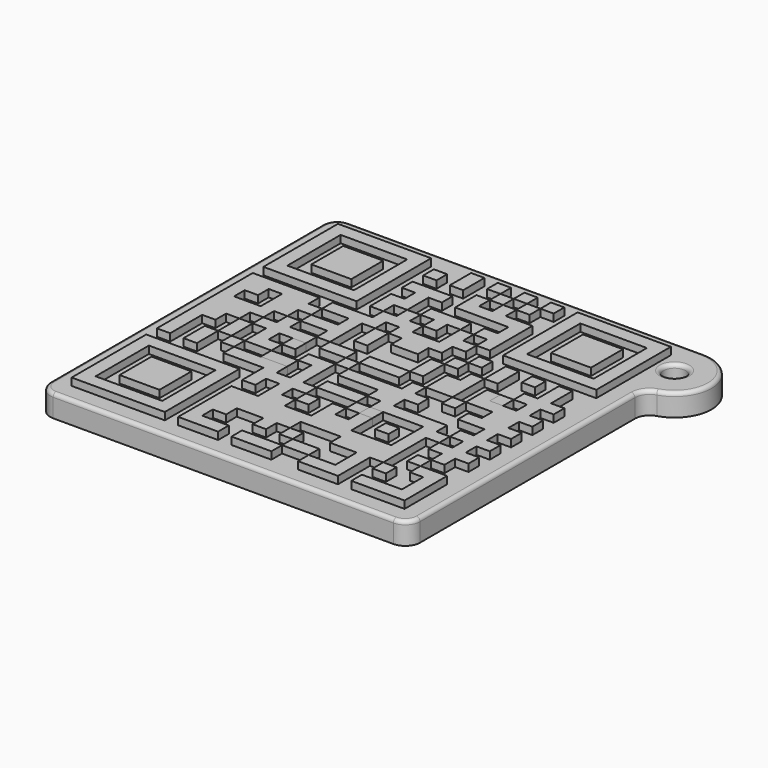
from build123d import *

# Parameters (mm, degrees)
F0_R     = 1.5
F1_DEPTH = 3
F2_R     = 2
F3_W     = 1.8
F3_H     = 1.8
F4_DEPTH = 1
F5_W     = 1.8
F5_H     = 1.8
F6_DEPTH = 1
F5_W_2   = 3.6
F7_R     = 0.5


with BuildPart() as f1:
    # F0 (on Top) → F1 (new body)
    with BuildSketch(Plane.XY):
        with BuildLine():
            Line((25, 25), (-25, 25))
            Line((-25, 25), (-25, -25))
            Line((-25, -25), (25, -25))
            Line((25, -25), (25, 15))
            ThreePointArc((25, 15), (30, 20), (25, 25))
        make_face()
        with Locations((25, 20)):
            Circle(F0_R, mode=Mode.SUBTRACT)
    extrude(amount=-F1_DEPTH)

    # F2
    f2_edges = [f1.edges().sort_by_distance(p)[0] for p in [
        (-25, -25, -1.5),
        (25, -25, -1.5),
        (25, 15, -1.5),
        (-25, 25, -1.5),
    ]]
    fillet(f2_edges, radius=F2_R)

    # F7
    f7_edges = [f1.edges().sort_by_distance(p)[0] for p in [
        (23.5, 20, 0),
        (23.5, 20, -3),
        (1, 25, 0),
    ]]
    fillet(f7_edges, radius=F7_R)


with BuildPart() as f4:
    # F3 (on Top) → F4 (new body)
    with BuildSketch(Plane.XY):
        with Locations((21.5957503378, 21.6023441762)):
            Rectangle(F3_W, F3_H)
        with Locations((21.5957503378, 19.8023441762)):
            Rectangle(F3_W, F3_H)
        with Locations((21.5957503378, 18.0023441762)):
            Rectangle(F3_W, F3_H)
        with Locations((21.5957503378, 16.2023441762)):
            Rectangle(F3_W, F3_H)
        with Locations((21.5957503378, 14.4023441762)):
            Rectangle(F3_W, F3_H)
        with Locations((21.5957503378, 12.6023441762)):
            Rectangle(F3_W, F3_H)
        with Locations((21.5957503378, 10.8023441762)):
            Rectangle(F3_W, F3_H)
        with Locations((19.7957503378, 21.6023441762)):
            Rectangle(F3_W, F3_H)
        with Locations((17.9957503378, 21.6023441762)):
            Rectangle(F3_W, F3_H)
        with Locations((16.1957503378, 21.6023441762)):
            Rectangle(F3_W, F3_H)
        with Locations((14.3957503378, 21.6023441762)):
            Rectangle(F3_W, F3_H)
        with Locations((12.5957503378, 21.6023441762)):
            Rectangle(F3_W, F3_H)
        with Locations((10.7957503378, 21.6023441762)):
            Rectangle(F3_W, F3_H)
        with Locations((10.7957503378, 19.8023441762)):
            Rectangle(F3_W, F3_H)
        with Locations((10.7957503378, 18.0023441762)):
            Rectangle(F3_W, F3_H)
        with Locations((10.7957503378, 16.2023441762)):
            Rectangle(F3_W, F3_H)
        with Locations((10.7957503378, 14.4023441762)):
            Rectangle(F3_W, F3_H)
        with Locations((10.7957503378, 12.6023441762)):
            Rectangle(F3_W, F3_H)
        with Locations((10.7957503378, 10.8023441762)):
            Rectangle(F3_W, F3_H)
        with Locations((12.5957503378, 10.8023441762)):
            Rectangle(F3_W, F3_H)
        with Locations((14.3957503378, 10.8023441762)):
            Rectangle(F3_W, F3_H)
        with Locations((16.1957503378, 10.8023441762)):
            Rectangle(F3_W, F3_H)
        with Locations((17.9957503378, 10.8023441762)):
            Rectangle(F3_W, F3_H)
        with Locations((19.7957503378, 10.8023441762)):
            Rectangle(F3_W, F3_H)
    extrude(amount=F4_DEPTH)


with BuildPart() as f4b:
    # F3 (on Top) → F4, piece 2 (new body)
    with BuildSketch(Plane.XY):
        with Locations((21.5957503378, -21.5976558238)):
            Rectangle(F3_W, F3_H)
        with Locations((21.5957503378, -16.1976558238)):
            Rectangle(F3_W, F3_H)
        with Locations((21.5957503378, -17.9976558238)):
            Rectangle(F3_W, F3_H)
        with Locations((21.5957503378, -19.7976558238)):
            Rectangle(F3_W, F3_H)
        with Locations((19.7957503378, -21.5976558238)):
            Rectangle(F3_W, F3_H)
        with Locations((17.9957503378, -21.5976558238)):
            Rectangle(F3_W, F3_H)
        with Locations((16.1957503378, -21.5976558238)):
            Rectangle(F3_W, F3_H)
        with Locations((19.7957503378, -16.1976558238)):
            Rectangle(F3_W, F3_H)
    extrude(amount=F4_DEPTH)


with BuildPart() as f4c:
    # F3 (on Top) → F4, piece 3 (new body)
    with BuildSketch(Plane.XY):
        with Locations((-21.6042496622, 21.6023441762)):
            Rectangle(F3_W, F3_H)
        with Locations((-10.8042496622, 21.6023441762)):
            Rectangle(F3_W, F3_H)
        with Locations((-12.6042496622, 21.6023441762)):
            Rectangle(F3_W, F3_H)
        with Locations((-14.4042496622, 21.6023441762)):
            Rectangle(F3_W, F3_H)
        with Locations((-16.2042496622, 21.6023441762)):
            Rectangle(F3_W, F3_H)
        with Locations((-18.0042496622, 21.6023441762)):
            Rectangle(F3_W, F3_H)
        with Locations((-19.8042496622, 21.6023441762)):
            Rectangle(F3_W, F3_H)
        with Locations((-21.6042496622, 19.8023441762)):
            Rectangle(F3_W, F3_H)
        with Locations((-21.6042496622, 18.0023441762)):
            Rectangle(F3_W, F3_H)
        with Locations((-21.6042496622, 16.2023441762)):
            Rectangle(F3_W, F3_H)
        with Locations((-21.6042496622, 14.4023441762)):
            Rectangle(F3_W, F3_H)
        with Locations((-21.6042496622, 12.6023441762)):
            Rectangle(F3_W, F3_H)
        with Locations((-21.6042496622, 10.8023441762)):
            Rectangle(F3_W, F3_H)
        with Locations((-19.8042496622, 10.8023441762)):
            Rectangle(F3_W, F3_H)
        with Locations((-18.0042496622, 10.8023441762)):
            Rectangle(F3_W, F3_H)
        with Locations((-16.2042496622, 10.8023441762)):
            Rectangle(F3_W, F3_H)
        with Locations((-14.4042496622, 10.8023441762)):
            Rectangle(F3_W, F3_H)
        with Locations((-12.6042496622, 10.8023441762)):
            Rectangle(F3_W, F3_H)
        with Locations((-10.8042496622, 10.8023441762)):
            Rectangle(F3_W, F3_H)
        with Locations((-10.8042496622, 12.6023441762)):
            Rectangle(F3_W, F3_H)
        with Locations((-10.8042496622, 14.4023441762)):
            Rectangle(F3_W, F3_H)
        with Locations((-10.8042496622, 16.2023441762)):
            Rectangle(F3_W, F3_H)
        with Locations((-10.8042496622, 18.0023441762)):
            Rectangle(F3_W, F3_H)
        with Locations((-10.8042496622, 19.8023441762)):
            Rectangle(F3_W, F3_H)
    extrude(amount=F4_DEPTH)


with BuildPart() as f4d:
    # F3 (on Top) → F4, piece 4 (new body)
    with BuildSketch(Plane.XY):
        with Locations((-21.6042496622, -21.5976558238)):
            Rectangle(F3_W, F3_H)
        with Locations((-10.8042496622, -21.5976558238)):
            Rectangle(F3_W, F3_H)
        with Locations((-12.6042496622, -21.5976558238)):
            Rectangle(F3_W, F3_H)
        with Locations((-14.4042496622, -21.5976558238)):
            Rectangle(F3_W, F3_H)
        with Locations((-16.2042496622, -21.5976558238)):
            Rectangle(F3_W, F3_H)
        with Locations((-18.0042496622, -21.5976558238)):
            Rectangle(F3_W, F3_H)
        with Locations((-19.8042496622, -21.5976558238)):
            Rectangle(F3_W, F3_H)
        with Locations((-21.6042496622, -10.7976558238)):
            Rectangle(F3_W, F3_H)
        with Locations((-21.6042496622, -12.5976558238)):
            Rectangle(F3_W, F3_H)
        with Locations((-21.6042496622, -14.3976558238)):
            Rectangle(F3_W, F3_H)
        with Locations((-21.6042496622, -16.1976558238)):
            Rectangle(F3_W, F3_H)
        with Locations((-21.6042496622, -17.9976558238)):
            Rectangle(F3_W, F3_H)
        with Locations((-21.6042496622, -19.7976558238)):
            Rectangle(F3_W, F3_H)
        with Locations((-19.8042496622, -10.7976558238)):
            Rectangle(F3_W, F3_H)
        with Locations((-18.0042496622, -10.7976558238)):
            Rectangle(F3_W, F3_H)
        with Locations((-16.2042496622, -10.7976558238)):
            Rectangle(F3_W, F3_H)
        with Locations((-14.4042496622, -10.7976558238)):
            Rectangle(F3_W, F3_H)
        with Locations((-12.6042496622, -10.7976558238)):
            Rectangle(F3_W, F3_H)
        with Locations((-10.8042496622, -10.7976558238)):
            Rectangle(F3_W, F3_H)
        with Locations((-10.8042496622, -12.5976558238)):
            Rectangle(F3_W, F3_H)
        with Locations((-10.8042496622, -14.3976558238)):
            Rectangle(F3_W, F3_H)
        with Locations((-10.8042496622, -16.1976558238)):
            Rectangle(F3_W, F3_H)
        with Locations((-10.8042496622, -17.9976558238)):
            Rectangle(F3_W, F3_H)
        with Locations((-10.8042496622, -19.7976558238)):
            Rectangle(F3_W, F3_H)
    extrude(amount=F4_DEPTH)


with BuildPart() as f4e:
    # F3 (on Top) → F4, piece 5 (new body)
    with BuildSketch(Plane.XY):
        with Locations((21.5957503378, 3.6023441762)):
            Rectangle(F3_W, F3_H)
        with Locations((21.5957503378, 0.0023441762)):
            Rectangle(F3_W, F3_H)
        with Locations((21.5957503378, -3.5976558238)):
            Rectangle(F3_W, F3_H)
        with Locations((21.5957503378, -7.1976558238)):
            Rectangle(F3_W, F3_H)
        with Locations((21.5957503378, -10.7976558238)):
            Rectangle(F3_W, F3_H)
        with Locations((19.7957503378, -12.5976558238)):
            Rectangle(F3_W, F3_H)
        with Locations((19.7957503378, -10.7976558238)):
            Rectangle(F3_W, F3_H)
        with Locations((19.7957503378, -8.9976558238)):
            Rectangle(F3_W, F3_H)
        with Locations((19.7957503378, -7.1976558238)):
            Rectangle(F3_W, F3_H)
        with Locations((19.7957503378, -5.3976558238)):
            Rectangle(F3_W, F3_H)
        with Locations((19.7957503378, -3.5976558238)):
            Rectangle(F3_W, F3_H)
        with Locations((17.9957503378, -10.7976558238)):
            Rectangle(F3_W, F3_H)
        with Locations((17.9957503378, -7.1976558238)):
            Rectangle(F3_W, F3_H)
        with Locations((16.1957503378, -3.5976558238)):
            Rectangle(F3_W, F3_H)
        with Locations((17.9957503378, -3.5976558238)):
            Rectangle(F3_W, F3_H)
        with Locations((17.9957503378, -1.7976558238)):
            Rectangle(F3_W, F3_H)
        with Locations((19.7957503378, -1.7976558238)):
            Rectangle(F3_W, F3_H)
        with Locations((19.7957503378, 7.2023441762)):
            Rectangle(F3_W, F3_H)
        with Locations((19.7957503378, 5.4023441762)):
            Rectangle(F3_W, F3_H)
        with Locations((19.7957503378, 3.6023441762)):
            Rectangle(F3_W, F3_H)
        with Locations((17.9957503378, 3.6023441762)):
            Rectangle(F3_W, F3_H)
        with Locations((19.7957503378, 1.8023441762)):
            Rectangle(F3_W, F3_H)
        with Locations((19.7957503378, 0.0023441762)):
            Rectangle(F3_W, F3_H)
        with Locations((17.9957503378, 0.0023441762)):
            Rectangle(F3_W, F3_H)
        with Locations((14.3957503378, 0.0023441762)):
            Rectangle(F3_W, F3_H)
        with Locations((16.1957503378, 0.0023441762)):
            Rectangle(F3_W, F3_H)
        with Locations((14.3957503378, 1.8023441762)):
            Rectangle(F3_W, F3_H)
    extrude(amount=F4_DEPTH)


with BuildPart() as f4f:
    # F3 (on Top) → F4, piece 6 (new body)
    with BuildSketch(Plane.XY):
        with Locations((12.5957503378, -21.5976558238)):
            Rectangle(F3_W, F3_H)
        with Locations((10.7957503378, -21.5976558238)):
            Rectangle(F3_W, F3_H)
        with Locations((8.9957503378, -21.5976558238)):
            Rectangle(F3_W, F3_H)
        with Locations((-3.6042496622, -21.5976558238)):
            Rectangle(F3_W, F3_H)
        with Locations((-5.4042496622, -21.5976558238)):
            Rectangle(F3_W, F3_H)
        with Locations((-7.2042496622, -21.5976558238)):
            Rectangle(F3_W, F3_H)
        with Locations((-12.6042496622, -7.1976558238)):
            Rectangle(F3_W, F3_H)
        with Locations((-10.8042496622, -7.1976558238)):
            Rectangle(F3_W, F3_H)
        with Locations((12.5957503378, -19.7976558238)):
            Rectangle(F3_W, F3_H)
        with Locations((12.5957503378, -17.9976558238)):
            Rectangle(F3_W, F3_H)
        with Locations((-7.2042496622, -19.7976558238)):
            Rectangle(F3_W, F3_H)
        with Locations((-7.2042496622, -17.9976558238)):
            Rectangle(F3_W, F3_H)
        with Locations((-5.4042496622, -17.9976558238)):
            Rectangle(F3_W, F3_H)
        with Locations((-0.0042496622, -17.9976558238)):
            Rectangle(F3_W, F3_H)
        with Locations((-7.2042496622, -16.1976558238)):
            Rectangle(F3_W, F3_H)
        with Locations((-5.4042496622, -16.1976558238)):
            Rectangle(F3_W, F3_H)
        with Locations((-3.6042496622, -16.1976558238)):
            Rectangle(F3_W, F3_H)
        with Locations((-1.8042496622, -16.1976558238)):
            Rectangle(F3_W, F3_H)
        with Locations((-0.0042496622, -16.1976558238)):
            Rectangle(F3_W, F3_H)
        with Locations((1.7957503378, -16.1976558238)):
            Rectangle(F3_W, F3_H)
        with Locations((8.9957503378, -16.1976558238)):
            Rectangle(F3_W, F3_H)
        with Locations((10.7957503378, -16.1976558238)):
            Rectangle(F3_W, F3_H)
        with Locations((12.5957503378, -16.1976558238)):
            Rectangle(F3_W, F3_H)
        with Locations((14.3957503378, -16.1976558238)):
            Rectangle(F3_W, F3_H)
        with Locations((14.3957503378, -7.1976558238)):
            Rectangle(F3_W, F3_H)
        with Locations((14.3957503378, -8.9976558238)):
            Rectangle(F3_W, F3_H)
        with Locations((16.1957503378, -8.9976558238)):
            Rectangle(F3_W, F3_H)
        with Locations((14.3957503378, -10.7976558238)):
            Rectangle(F3_W, F3_H)
        with Locations((14.3957503378, -12.5976558238)):
            Rectangle(F3_W, F3_H)
        with Locations((14.3957503378, -14.3976558238)):
            Rectangle(F3_W, F3_H)
        with Locations((12.5957503378, -14.3976558238)):
            Rectangle(F3_W, F3_H)
        with Locations((10.7957503378, -14.3976558238)):
            Rectangle(F3_W, F3_H)
        with Locations((8.9957503378, -14.3976558238)):
            Rectangle(F3_W, F3_H)
        with Locations((-7.2042496622, -14.3976558238)):
            Rectangle(F3_W, F3_H)
        with Locations((-5.4042496622, -14.3976558238)):
            Rectangle(F3_W, F3_H)
        with Locations((-3.6042496622, -14.3976558238)):
            Rectangle(F3_W, F3_H)
        with Locations((-1.8042496622, -14.3976558238)):
            Rectangle(F3_W, F3_H)
        with Locations((-0.0042496622, -14.3976558238)):
            Rectangle(F3_W, F3_H)
        with Locations((1.7957503378, -14.3976558238)):
            Rectangle(F3_W, F3_H)
        with Locations((3.5957503378, -14.3976558238)):
            Rectangle(F3_W, F3_H)
        with Locations((5.3957503378, -14.3976558238)):
            Rectangle(F3_W, F3_H)
        with Locations((7.1957503378, -14.3976558238)):
            Rectangle(F3_W, F3_H)
        with Locations((7.1957503378, -12.5976558238)):
            Rectangle(F3_W, F3_H)
        with Locations((5.3957503378, -12.5976558238)):
            Rectangle(F3_W, F3_H)
        with Locations((3.5957503378, -12.5976558238)):
            Rectangle(F3_W, F3_H)
        with Locations((-1.8042496622, -12.5976558238)):
            Rectangle(F3_W, F3_H)
        with Locations((-3.6042496622, -12.5976558238)):
            Rectangle(F3_W, F3_H)
        with Locations((-7.2042496622, -10.7976558238)):
            Rectangle(F3_W, F3_H)
        with Locations((-3.6042496622, -10.7976558238)):
            Rectangle(F3_W, F3_H)
        with Locations((3.5957503378, -10.7976558238)):
            Rectangle(F3_W, F3_H)
        with Locations((7.1957503378, -10.7976558238)):
            Rectangle(F3_W, F3_H)
        with Locations((-7.2042496622, -8.9976558238)):
            Rectangle(F3_W, F3_H)
        with Locations((-5.4042496622, -8.9976558238)):
            Rectangle(F3_W, F3_H)
        with Locations((-3.6042496622, -8.9976558238)):
            Rectangle(F3_W, F3_H)
        with Locations((-1.8042496622, -8.9976558238)):
            Rectangle(F3_W, F3_H)
        with Locations((-5.4042496622, -3.5976558238)):
            Rectangle(F3_W, F3_H)
        with Locations((-3.6042496622, -3.5976558238)):
            Rectangle(F3_W, F3_H)
        with Locations((-3.6042496622, -5.3976558238)):
            Rectangle(F3_W, F3_H)
        with Locations((-3.6042496622, -7.1976558238)):
            Rectangle(F3_W, F3_H)
        with Locations((-0.0042496622, -3.5976558238)):
            Rectangle(F3_W, F3_H)
        with Locations((1.7957503378, -3.5976558238)):
            Rectangle(F3_W, F3_H)
        with Locations((3.5957503378, -3.5976558238)):
            Rectangle(F3_W, F3_H)
        with Locations((5.3957503378, -3.5976558238)):
            Rectangle(F3_W, F3_H)
        with Locations((8.9957503378, -3.5976558238)):
            Rectangle(F3_W, F3_H)
        with Locations((5.3957503378, -5.3976558238)):
            Rectangle(F3_W, F3_H)
        with Locations((7.1957503378, -5.3976558238)):
            Rectangle(F3_W, F3_H)
        with Locations((7.1957503378, -3.5976558238)):
            Rectangle(F3_W, F3_H)
        with Locations((7.1957503378, -1.7976558238)):
            Rectangle(F3_W, F3_H)
        with Locations((7.1957503378, -7.1976558238)):
            Rectangle(F3_W, F3_H)
        with Locations((8.9957503378, -7.1976558238)):
            Rectangle(F3_W, F3_H)
        with Locations((10.7957503378, -7.1976558238)):
            Rectangle(F3_W, F3_H)
        with Locations((12.5957503378, -7.1976558238)):
            Rectangle(F3_W, F3_H)
        with Locations((-7.2042496622, -7.1976558238)):
            Rectangle(F3_W, F3_H)
        with Locations((-9.0042496622, -7.1976558238)):
            Rectangle(F3_W, F3_H)
    extrude(amount=F4_DEPTH)


with BuildPart() as f4g:
    # F3 (on Top) → F4, piece 7 (new body)
    with BuildSketch(Plane.XY):
        with Locations((3.5957503378, -21.5976558238)):
            Rectangle(F3_W, F3_H)
        with Locations((1.7957503378, -21.5976558238)):
            Rectangle(F3_W, F3_H)
        with Locations((-0.0042496622, -21.5976558238)):
            Rectangle(F3_W, F3_H)
    extrude(amount=F4_DEPTH)


with BuildPart() as f4h:
    # F3 (on Top) → F4, piece 8 (new body)
    with BuildSketch(Plane.XY):
        with Locations((-3.6042496622, 21.6023441762)):
            Rectangle(F3_W, F3_H)
        with Locations((-3.6042496622, 19.8023441762)):
            Rectangle(F3_W, F3_H)
    extrude(amount=F4_DEPTH)


with BuildPart() as f4i:
    # F3 (on Top) → F4, piece 9 (new body)
    with BuildSketch(Plane.XY):
        with Locations((-21.6042496622, 7.2023441762)):
            Rectangle(F3_W, F3_H)
        with Locations((-21.6042496622, 5.4023441762)):
            Rectangle(F3_W, F3_H)
        with Locations((-21.6042496622, 3.6023441762)):
            Rectangle(F3_W, F3_H)
        with Locations((-21.6042496622, 1.8023441762)):
            Rectangle(F3_W, F3_H)
        with Locations((-21.6042496622, 0.0023441762)):
            Rectangle(F3_W, F3_H)
        with Locations((-21.6042496622, -1.7976558238)):
            Rectangle(F3_W, F3_H)
        with Locations((-21.6042496622, -3.5976558238)):
            Rectangle(F3_W, F3_H)
        with Locations((-21.6042496622, -5.3976558238)):
            Rectangle(F3_W, F3_H)
        with Locations((-21.6042496622, -7.1976558238)):
            Rectangle(F3_W, F3_H)
        with Locations((-19.8042496622, -1.7976558238)):
            Rectangle(F3_W, F3_H)
        with Locations((-19.8042496622, 0.0023441762)):
            Rectangle(F3_W, F3_H)
        with Locations((-19.8042496622, 1.8023441762)):
            Rectangle(F3_W, F3_H)
        with Locations((-18.0042496622, 0.0023441762)):
            Rectangle(F3_W, F3_H)
        with Locations((-18.0042496622, 1.8023441762)):
            Rectangle(F3_W, F3_H)
        with Locations((-16.2042496622, 1.8023441762)):
            Rectangle(F3_W, F3_H)
        with Locations((-12.6042496622, 5.4023441762)):
            Rectangle(F3_W, F3_H)
        with Locations((-14.4042496622, 5.4023441762)):
            Rectangle(F3_W, F3_H)
        with Locations((-16.2042496622, 5.4023441762)):
            Rectangle(F3_W, F3_H)
        with Locations((-14.4042496622, 7.2023441762)):
            Rectangle(F3_W, F3_H)
        with Locations((-19.8042496622, 5.4023441762)):
            Rectangle(F3_W, F3_H)
        with Locations((-19.8042496622, 7.2023441762)):
            Rectangle(F3_W, F3_H)
        with Locations((-18.0042496622, 7.2023441762)):
            Rectangle(F3_W, F3_H)
        with Locations((-16.2042496622, 7.2023441762)):
            Rectangle(F3_W, F3_H)
        with Locations((-16.2042496622, 3.6023441762)):
            Rectangle(F3_W, F3_H)
        with Locations((-14.4042496622, 3.6023441762)):
            Rectangle(F3_W, F3_H)
    extrude(amount=F4_DEPTH)


with BuildPart() as f4j:
    # F3 (on Top) → F4, piece 10 (new body)
    with BuildSketch(Plane.XY):
        with Locations((-18.0042496622, 18.0023441762)):
            Rectangle(F3_W, F3_H)
        with Locations((-16.2042496622, 18.0023441762)):
            Rectangle(F3_W, F3_H)
        with Locations((-14.4042496622, 18.0023441762)):
            Rectangle(F3_W, F3_H)
        with Locations((-14.4042496622, 16.2023441762)):
            Rectangle(F3_W, F3_H)
        with Locations((-14.4042496622, 14.4023441762)):
            Rectangle(F3_W, F3_H)
        with Locations((-16.2042496622, 14.4023441762)):
            Rectangle(F3_W, F3_H)
        with Locations((-18.0042496622, 14.4023441762)):
            Rectangle(F3_W, F3_H)
        with Locations((-18.0042496622, 16.2023441762)):
            Rectangle(F3_W, F3_H)
        with Locations((-16.2042496622, 16.2023441762)):
            Rectangle(F3_W, F3_H)
    extrude(amount=F4_DEPTH)


with BuildPart() as f4k:
    # F3 (on Top) → F4, piece 11 (new body)
    with BuildSketch(Plane.XY):
        with Locations((-7.2042496622, 19.8023441762)):
            Rectangle(F3_W, F3_H)
    extrude(amount=F4_DEPTH)


with BuildPart() as f4l:
    # F3 (on Top) → F4, piece 12 (new body)
    with BuildSketch(Plane.XY):
        with Locations((-7.2042496622, 16.2023441762)):
            Rectangle(F3_W, F3_H)
        with Locations((-5.4042496622, 16.2023441762)):
            Rectangle(F3_W, F3_H)
        with Locations((-3.6042496622, 16.2023441762)):
            Rectangle(F3_W, F3_H)
        with Locations((-5.4042496622, 14.4023441762)):
            Rectangle(F3_W, F3_H)
        with Locations((-5.4042496622, 12.6023441762)):
            Rectangle(F3_W, F3_H)
        with Locations((-7.2042496622, 12.6023441762)):
            Rectangle(F3_W, F3_H)
        with Locations((-7.2042496622, 10.8023441762)):
            Rectangle(F3_W, F3_H)
    extrude(amount=F4_DEPTH)


with BuildPart() as f4m:
    # F3 (on Top) → F4, piece 13 (new body)
    with BuildSketch(Plane.XY):
        with Locations((14.3957503378, 14.4023441762)):
            Rectangle(F3_W, F3_H)
        with Locations((14.3957503378, 16.2023441762)):
            Rectangle(F3_W, F3_H)
        with Locations((14.3957503378, 18.0023441762)):
            Rectangle(F3_W, F3_H)
        with Locations((16.1957503378, 18.0023441762)):
            Rectangle(F3_W, F3_H)
        with Locations((16.1957503378, 16.2023441762)):
            Rectangle(F3_W, F3_H)
        with Locations((16.1957503378, 14.4023441762)):
            Rectangle(F3_W, F3_H)
        with Locations((17.9957503378, 14.4023441762)):
            Rectangle(F3_W, F3_H)
        with Locations((17.9957503378, 16.2023441762)):
            Rectangle(F3_W, F3_H)
        with Locations((17.9957503378, 18.0023441762)):
            Rectangle(F3_W, F3_H)
    extrude(amount=F4_DEPTH)


with BuildPart() as f4n:
    # F3 (on Top) → F4, piece 14 (new body)
    with BuildSketch(Plane.XY):
        with Locations((-0.0042496622, 21.6023441762)):
            Rectangle(F3_W, F3_H)
    extrude(amount=F4_DEPTH)


with BuildPart() as f4o:
    # F3 (on Top) → F4, piece 15 (new body)
    with BuildSketch(Plane.XY):
        with Locations((3.5957503378, 21.6023441762)):
            Rectangle(F3_W, F3_H)
    extrude(amount=F4_DEPTH)


with BuildPart() as f4p:
    # F3 (on Top) → F4, piece 16 (new body)
    with BuildSketch(Plane.XY):
        with Locations((7.1957503378, 21.6023441762)):
            Rectangle(F3_W, F3_H)
    extrude(amount=F4_DEPTH)


with BuildPart() as f4q:
    # F3 (on Top) → F4, piece 17 (new body)
    with BuildSketch(Plane.XY):
        with Locations((1.7957503378, 19.8023441762)):
            Rectangle(F3_W, F3_H)
    extrude(amount=F4_DEPTH)


with BuildPart() as f4r:
    # F3 (on Top) → F4, piece 18 (new body)
    with BuildSketch(Plane.XY):
        with Locations((5.3957503378, 19.8023441762)):
            Rectangle(F3_W, F3_H)
    extrude(amount=F4_DEPTH)


with BuildPart() as f4s:
    # F3 (on Top) → F4, piece 19 (new body)
    with BuildSketch(Plane.XY):
        with Locations((-0.0042496622, 18.0023441762)):
            Rectangle(F3_W, F3_H)
        with Locations((-0.0042496622, 16.2023441762)):
            Rectangle(F3_W, F3_H)
        with Locations((1.7957503378, 16.2023441762)):
            Rectangle(F3_W, F3_H)
        with Locations((3.5957503378, 16.2023441762)):
            Rectangle(F3_W, F3_H)
        with Locations((3.5957503378, 18.0023441762)):
            Rectangle(F3_W, F3_H)
        with Locations((5.3957503378, 16.2023441762)):
            Rectangle(F3_W, F3_H)
        with Locations((7.1957503378, 16.2023441762)):
            Rectangle(F3_W, F3_H)
        with Locations((7.1957503378, 14.4023441762)):
            Rectangle(F3_W, F3_H)
        with Locations((7.1957503378, 12.6023441762)):
            Rectangle(F3_W, F3_H)
        with Locations((7.1957503378, 10.8023441762)):
            Rectangle(F3_W, F3_H)
        with Locations((5.3957503378, 12.6023441762)):
            Rectangle(F3_W, F3_H)
    extrude(amount=F4_DEPTH)


with BuildPart() as f4t:
    # F3 (on Top) → F4, piece 20 (new body)
    with BuildSketch(Plane.XY):
        with Locations((-1.8042496622, 12.6023441762)):
            Rectangle(F3_W, F3_H)
        with Locations((-0.0042496622, 12.6023441762)):
            Rectangle(F3_W, F3_H)
        with Locations((1.7957503378, 12.6023441762)):
            Rectangle(F3_W, F3_H)
        with Locations((-0.0042496622, 10.8023441762)):
            Rectangle(F3_W, F3_H)
    extrude(amount=F4_DEPTH)


with BuildPart() as f4u:
    # F3 (on Top) → F4, piece 21 (new body)
    with BuildSketch(Plane.XY):
        with Locations((3.5957503378, 10.8023441762)):
            Rectangle(F3_W, F3_H)
        with Locations((3.5957503378, 9.0023441762)):
            Rectangle(F3_W, F3_H)
        with Locations((3.5957503378, 7.2023441762)):
            Rectangle(F3_W, F3_H)
        with Locations((5.3957503378, 9.0023441762)):
            Rectangle(F3_W, F3_H)
        with Locations((1.7957503378, 5.4023441762)):
            Rectangle(F3_W, F3_H)
        with Locations((1.7957503378, 7.2023441762)):
            Rectangle(F3_W, F3_H)
        with Locations((-0.0042496622, 7.2023441762)):
            Rectangle(F3_W, F3_H)
        with Locations((-0.0042496622, 5.4023441762)):
            Rectangle(F3_W, F3_H)
        with Locations((-1.8042496622, 9.0023441762)):
            Rectangle(F3_W, F3_H)
        with Locations((-3.6042496622, 9.0023441762)):
            Rectangle(F3_W, F3_H)
        with Locations((-3.6042496622, 10.8023441762)):
            Rectangle(F3_W, F3_H)
        with Locations((-5.4042496622, 9.0023441762)):
            Rectangle(F3_W, F3_H)
        with Locations((-5.4042496622, 7.2023441762)):
            Rectangle(F3_W, F3_H)
        with Locations((-7.2042496622, 7.2023441762)):
            Rectangle(F3_W, F3_H)
        with Locations((-9.0042496622, 7.2023441762)):
            Rectangle(F3_W, F3_H)
        with Locations((-10.8042496622, 7.2023441762)):
            Rectangle(F3_W, F3_H)
        with Locations((-7.2042496622, 5.4023441762)):
            Rectangle(F3_W, F3_H)
        with Locations((-7.2042496622, 3.6023441762)):
            Rectangle(F3_W, F3_H)
        with Locations((-7.2042496622, 1.8023441762)):
            Rectangle(F3_W, F3_H)
        with Locations((-9.0042496622, 3.6023441762)):
            Rectangle(F3_W, F3_H)
        with Locations((-10.8042496622, 3.6023441762)):
            Rectangle(F3_W, F3_H)
        with Locations((-1.8042496622, 7.2023441762)):
            Rectangle(F3_W, F3_H)
    extrude(amount=F4_DEPTH)


with BuildPart() as f4v:
    # F3 (on Top) → F4, piece 22 (new body)
    with BuildSketch(Plane.XY):
        with Locations((-3.6042496622, 3.6023441762)):
            Rectangle(F3_W, F3_H)
        with Locations((-3.6042496622, 5.4023441762)):
            Rectangle(F3_W, F3_H)
    extrude(amount=F4_DEPTH)


with BuildPart() as f4w:
    # F3 (on Top) → F4, piece 23 (new body)
    with BuildSketch(Plane.XY):
        with Locations((-18.0042496622, -14.3976558238)):
            Rectangle(F3_W, F3_H)
        with Locations((-16.2042496622, -14.3976558238)):
            Rectangle(F3_W, F3_H)
        with Locations((-14.4042496622, -14.3976558238)):
            Rectangle(F3_W, F3_H)
        with Locations((-14.4042496622, -16.1976558238)):
            Rectangle(F3_W, F3_H)
        with Locations((-16.2042496622, -16.1976558238)):
            Rectangle(F3_W, F3_H)
        with Locations((-18.0042496622, -16.1976558238)):
            Rectangle(F3_W, F3_H)
        with Locations((-18.0042496622, -17.9976558238)):
            Rectangle(F3_W, F3_H)
        with Locations((-16.2042496622, -17.9976558238)):
            Rectangle(F3_W, F3_H)
        with Locations((-14.4042496622, -17.9976558238)):
            Rectangle(F3_W, F3_H)
    extrude(amount=F4_DEPTH)


with BuildPart() as f4x:
    # F3 (on Top) → F4, piece 24 (new body)
    with BuildSketch(Plane.XY):
        with Locations((-18.0042496622, -7.1976558238)):
            Rectangle(F3_W, F3_H)
        with Locations((-18.0042496622, -5.3976558238)):
            Rectangle(F3_W, F3_H)
    extrude(amount=F4_DEPTH)


with BuildPart() as f4y:
    # F3 (on Top) → F4, piece 25 (new body)
    with BuildSketch(Plane.XY):
        with Locations((-16.2042496622, -3.5976558238)):
            Rectangle(F3_W, F3_H)
        with Locations((-16.2042496622, -1.7976558238)):
            Rectangle(F3_W, F3_H)
    extrude(amount=F4_DEPTH)


with BuildPart() as f4z:
    # F3 (on Top) → F4, piece 26 (new body)
    with BuildSketch(Plane.XY):
        with Locations((-14.4042496622, -5.3976558238)):
            Rectangle(F3_W, F3_H)
    extrude(amount=F4_DEPTH)


with BuildPart() as f4ba:
    # F3 (on Top) → F4, piece 27 (new body)
    with BuildSketch(Plane.XY):
        with Locations((-10.8042496622, -3.5976558238)):
            Rectangle(F3_W, F3_H)
        with Locations((-12.6042496622, -3.5976558238)):
            Rectangle(F3_W, F3_H)
        with Locations((-12.6042496622, -1.7976558238)):
            Rectangle(F3_W, F3_H)
        with Locations((-14.4042496622, 0.0023441762)):
            Rectangle(F3_W, F3_H)
        with Locations((-12.6042496622, 0.0023441762)):
            Rectangle(F3_W, F3_H)
        with Locations((-12.6042496622, 1.8023441762)):
            Rectangle(F3_W, F3_H)
        with Locations((-10.8042496622, 0.0023441762)):
            Rectangle(F3_W, F3_H)
        with Locations((-9.0042496622, 0.0023441762)):
            Rectangle(F3_W, F3_H)
    extrude(amount=F4_DEPTH)


with BuildPart() as f4bb:
    # F3 (on Top) → F4, piece 28 (new body)
    with BuildSketch(Plane.XY):
        with Locations((17.9957503378, -14.3976558238)):
            Rectangle(F3_W, F3_H)
    extrude(amount=F4_DEPTH)


with BuildPart() as f4bc:
    # F3 (on Top) → F4, piece 29 (new body)
    with BuildSketch(Plane.XY):
        with Locations((16.1957503378, -17.9976558238)):
            Rectangle(F3_W, F3_H)
    extrude(amount=F4_DEPTH)


with BuildPart() as f4bd:
    # F3 (on Top) → F4, piece 30 (new body)
    with BuildSketch(Plane.XY):
        with Locations((16.1957503378, 7.2023441762)):
            Rectangle(F3_W, F3_H)
    extrude(amount=F4_DEPTH)


with BuildPart() as f4be:
    # F3 (on Top) → F4, piece 31 (new body)
    with BuildSketch(Plane.XY):
        with Locations((12.5957503378, 7.2023441762)):
            Rectangle(F3_W, F3_H)
        with Locations((12.5957503378, 5.4023441762)):
            Rectangle(F3_W, F3_H)
    extrude(amount=F4_DEPTH)


with BuildPart() as f4bf:
    # F3 (on Top) → F4, piece 32 (new body)
    with BuildSketch(Plane.XY):
        with Locations((8.9957503378, 7.2023441762)):
            Rectangle(F3_W, F3_H)
    extrude(amount=F4_DEPTH)


with BuildPart() as f4bg:
    # F3 (on Top) → F4, piece 33 (new body)
    with BuildSketch(Plane.XY):
        with Locations((7.1957503378, 5.4023441762)):
            Rectangle(F3_W, F3_H)
    extrude(amount=F4_DEPTH)


with BuildPart() as f4bh:
    # F3 (on Top) → F4, piece 34 (new body)
    with BuildSketch(Plane.XY):
        with Locations((5.3957503378, 3.6023441762)):
            Rectangle(F3_W, F3_H)
        with Locations((5.3957503378, 1.8023441762)):
            Rectangle(F3_W, F3_H)
    extrude(amount=F4_DEPTH)


with BuildPart() as f4bi:
    # F3 (on Top) → F4, piece 35 (new body)
    with BuildSketch(Plane.XY):
        with Locations((7.1957503378, -19.7976558238)):
            Rectangle(F3_W, F3_H)
        with Locations((5.3957503378, -19.7976558238)):
            Rectangle(F3_W, F3_H)
    extrude(amount=F4_DEPTH)


with BuildPart() as f4bj:
    # F3 (on Top) → F4, piece 36 (new body)
    with BuildSketch(Plane.XY):
        with Locations((3.5957503378, -17.9976558238)):
            Rectangle(F3_W, F3_H)
    extrude(amount=F4_DEPTH)


with BuildPart() as f4bk:
    # F3 (on Top) → F4, piece 37 (new body)
    with BuildSketch(Plane.XY):
        with Locations((-5.4042496622, 0.0023441762)):
            Rectangle(F3_W, F3_H)
        with Locations((-3.6042496622, 0.0023441762)):
            Rectangle(F3_W, F3_H)
    extrude(amount=F4_DEPTH)


with BuildPart() as f4bl:
    # F3 (on Top) → F4, piece 38 (new body)
    with BuildSketch(Plane.XY):
        with Locations((-1.8042496622, -1.7976558238)):
            Rectangle(F3_W, F3_H)
    extrude(amount=F4_DEPTH)


with BuildPart() as f4bm:
    # F3 (on Top) → F4, piece 39 (new body)
    with BuildSketch(Plane.XY):
        with Locations((-0.0042496622, 0.0023441762)):
            Rectangle(F3_W, F3_H)
        with Locations((1.7957503378, 0.0023441762)):
            Rectangle(F3_W, F3_H)
        with Locations((3.5957503378, 0.0023441762)):
            Rectangle(F3_W, F3_H)
    extrude(amount=F4_DEPTH)


with BuildPart() as f4bn:
    # F3 (on Top) → F4, piece 40 (new body)
    with BuildSketch(Plane.XY):
        with Locations((12.5957503378, -1.7976558238)):
            Rectangle(F3_W, F3_H)
    extrude(amount=F4_DEPTH)


with BuildPart() as f4bo:
    # F3 (on Top) → F4, piece 41 (new body)
    with BuildSketch(Plane.XY):
        with Locations((10.7957503378, -10.7976558238)):
            Rectangle(F3_W, F3_H)
    extrude(amount=F4_DEPTH)


with BuildPart() as f4bp:
    # F3 (on Top) → F4, piece 42 (new body)
    with BuildSketch(Plane.XY):
        with Locations((-0.0042496622, -10.7976558238)):
            Rectangle(F3_W, F3_H)
    extrude(amount=F4_DEPTH)


with BuildPart() as f4bq:
    # F3 (on Top) → F4, piece 43 (new body)
    with BuildSketch(Plane.XY):
        with Locations((-0.0042496622, -7.1976558238)):
            Rectangle(F3_W, F3_H)
        with Locations((1.7957503378, -7.1976558238)):
            Rectangle(F3_W, F3_H)
        with Locations((3.5957503378, -7.1976558238)):
            Rectangle(F3_W, F3_H)
    extrude(amount=F4_DEPTH)


with BuildPart() as f4br:
    # F3 (on Top) → F4, piece 44 (new body)
    with BuildSketch(Plane.XY):
        with Locations((5.3957503378, -8.9976558238)):
            Rectangle(F3_W, F3_H)
    extrude(amount=F4_DEPTH)


with BuildPart() as f4bs:
    # F3 (on Top) → F4, piece 45 (new body)
    with BuildSketch(Plane.XY):
        with Locations((8.9957503378, 0.0023441762)):
            Rectangle(F3_W, F3_H)
        with Locations((10.7957503378, 0.0023441762)):
            Rectangle(F3_W, F3_H)
        with Locations((10.7957503378, 1.8023441762)):
            Rectangle(F3_W, F3_H)
        with Locations((8.9957503378, 1.8023441762)):
            Rectangle(F3_W, F3_H)
        with Locations((10.7957503378, 3.6023441762)):
            Rectangle(F3_W, F3_H)
    extrude(amount=F4_DEPTH)


with BuildPart() as f6:
    # F5 (on Top) → F6 (new body)
    with BuildSketch(Plane.XY):
        with Locations((-9.0042496622, -1.7976558238)):
            Rectangle(F5_W, F5_H)
    extrude(amount=F6_DEPTH)


with BuildPart() as f6b:
    # F5 (on Top) → F6, piece 2 (new body)
    with BuildSketch(Plane.XY):
        with Locations((-8.1042496622, -5.3976558238)):
            Rectangle(F5_W_2, F5_H)
    extrude(amount=F6_DEPTH)


with BuildPart() as f6c:
    # F5 (on Top) → F6, piece 3 (new body)
    with BuildSketch(Plane.XY):
        with Locations((7.1957503378, -8.9976558238)):
            Rectangle(F5_W, F5_H)
    extrude(amount=F6_DEPTH)


with BuildPart() as f6d:
    # F5 (on Top) → F6, piece 4 (new body)
    with BuildSketch(Plane.XY):
        with Locations((16.1957503378, 1.8023441762)):
            Rectangle(F5_W, F5_H)
    extrude(amount=F6_DEPTH)


solid = Compound([f1.part, f4.part, f4b.part, f4c.part, f4d.part, f4e.part, f4f.part, f4g.part, f4h.part, f4i.part, f4j.part, f4k.part, f4l.part, f4m.part, f4n.part, f4o.part, f4p.part, f4q.part, f4r.part, f4s.part, f4t.part, f4u.part, f4v.part, f4w.part, f4x.part, f4y.part, f4z.part, f4ba.part, f4bb.part, f4bc.part, f4bd.part, f4be.part, f4bf.part, f4bg.part, f4bh.part, f4bi.part, f4bj.part, f4bk.part, f4bl.part, f4bm.part, f4bn.part, f4bo.part, f4bp.part, f4bq.part, f4br.part, f4bs.part, f6.part, f6b.part, f6c.part, f6d.part])
